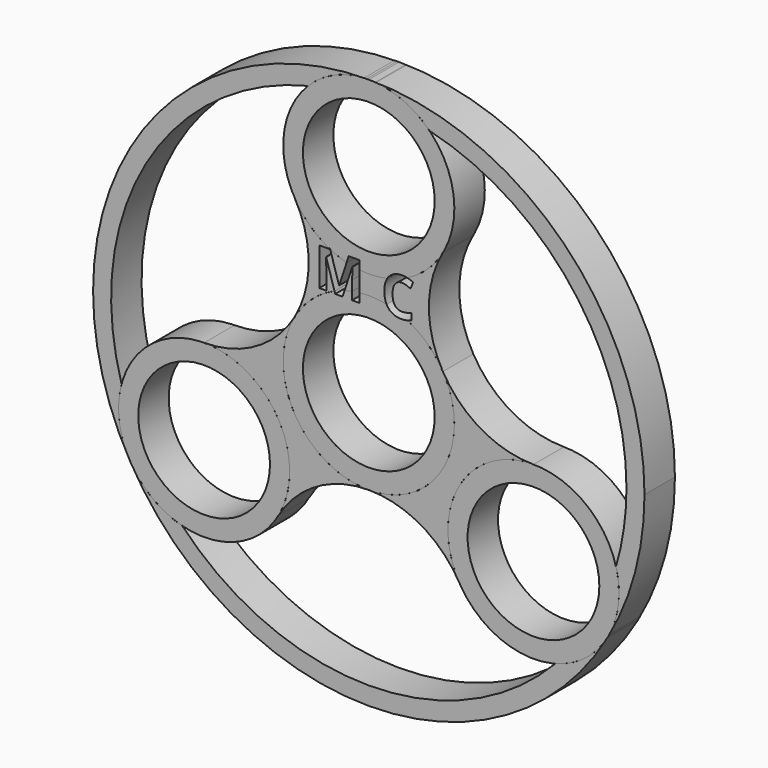
from build123d import *

# Parameters (mm, degrees)
F0_R         = 14.2875
F0_R_2       = 10.9982
F2_DEPTH     = 6.35
F3_TEXT_SIZE = 8.8194444444
F4_DEPTH     = 25.4


# Not quite as in the source:
# - Text() gives the source's letters only with a copy of the font that has no kerning and outlines rounded to 1/6400 em; it was checked with that copy


with BuildPart() as f2:
    # F0 (on Front) → F2 (new body)
    with BuildSketch(Plane.XZ):
        with Locations((0, 31.75)):
            Circle(F0_R)
        with Locations((0, 31.75)):
            Circle(F0_R_2, mode=Mode.SUBTRACT)
    extrude(amount=F2_DEPTH)


with BuildPart() as f2b:
    # F0 (on Front) → F2, piece 2 (new body)
    with BuildSketch(Plane.XZ):
        Circle(F0_R)
        Circle(F0_R_2, mode=Mode.SUBTRACT)
    extrude(amount=F2_DEPTH)


with BuildPart() as f2c:
    # F0 (on Front) → F2, piece 3 (new body)
    with BuildSketch(Plane.XZ):
        with Locations((-27.4963065702, -15.875)):
            Circle(F0_R)
        with Locations((-27.4963065702, -15.875)):
            Circle(F0_R_2, mode=Mode.SUBTRACT)
    extrude(amount=F2_DEPTH)


with BuildPart() as f2d:
    # F0 (on Front) → F2, piece 4 (new body)
    with BuildSketch(Plane.XZ):
        with Locations((27.4963065702, -15.875)):
            Circle(F0_R)
        with Locations((27.4963065702, -15.875)):
            Circle(F0_R_2, mode=Mode.SUBTRACT)
    extrude(amount=F2_DEPTH)


with BuildPart() as f2e:
    # F1 (on Front) → F2, piece 5 (new body)
    with BuildSketch(Plane.XZ):
        with BuildLine():
            ThreePointArc((12.3733379566, 24.60625), (0, 17.4625), (-12.3733379566, 24.60625))
            ThreePointArc((-12.3733379566, 24.60625), (-10.0338065702, 15.8750000272), (-12.3733379294, 7.1437500471))
            ThreePointArc((-12.3733379294, 7.1437500471), (-1.17e-08, 14.2875), (12.3733379177, 7.1437500674))
            ThreePointArc((12.3733379177, 7.1437500674), (10.0338065702, 15.8750000389), (12.3733379566, 24.60625))
        make_face()
    extrude(amount=F2_DEPTH)


with BuildPart() as f2f:
    # F1 (on Front) → F2, piece 6 (new body)
    with BuildSketch(Plane.XZ):
        with BuildLine():
            ThreePointArc((1.61e-08, -14.2875), (-12.3733379662, -7.1437499834), (-12.3733379294, 7.1437500471))
            ThreePointArc((-12.3733379294, 7.1437500471), (-18.7650565466, 0.7520314), (-27.4963065702, -1.5875))
            ThreePointArc((-27.4963065702, -1.5875), (-17.393518434, -5.7722118638), (-13.2088065702, -15.875))
            ThreePointArc((-13.2088065702, -15.875), (-13.6956413271, -19.5728771069), (-15.1229686136, -23.01875))
            ThreePointArc((-15.1229686136, -23.01875), (-8.731249993, -16.6270313824), (1.61e-08, -14.2875))
        make_face()
    extrude(amount=F2_DEPTH)


with BuildPart() as f2g:
    # F1 (on Front) → F2, piece 7 (new body)
    with BuildSketch(Plane.XZ):
        with BuildLine():
            ThreePointArc((27.4963065702, -1.5875), (18.7650565365, 0.7520314059), (12.3733379177, 7.1437500674))
            ThreePointArc((12.3733379177, 7.1437500674), (13.800665233, 3.6978771445), (14.2875, 0))
            ThreePointArc((14.2875, 0), (10.1027881419, -10.1027881305), (1.61e-08, -14.2875))
            ThreePointArc((1.61e-08, -14.2875), (8.731250007, -16.6270313904), (15.1229686136, -23.01875))
            ThreePointArc((15.1229686136, -23.01875), (15.1229686136, -8.73125), (27.4963065702, -1.5875))
        make_face()
    extrude(amount=F2_DEPTH)


with BuildPart() as f2h:
    # F1 (on Front) → F2, piece 8 (new body)
    with BuildSketch(Plane.XZ):
        with BuildLine():
            ThreePointArc((-31.1385341366, -29.6904563661), (-36.1711264704, -27.2275396255), (-39.8696444605, -23.0187501146))
            ThreePointArc((-39.8696444605, -23.0187501146), (0, -46.0375), (39.8696444605, -23.0187501146))
            ThreePointArc((39.8696444605, -23.0187501146), (36.1711264704, -27.2275396255), (31.1385341366, -29.6904563661))
            ThreePointArc((31.1385341366, -29.6904563661), (0, -43.024777831), (-31.1385341366, -29.6904563661))
        make_face()
    extrude(amount=F2_DEPTH)


with BuildPart() as f2i:
    # F1 (on Front) → F2, piece 9 (new body)
    with BuildSketch(Plane.XZ):
        with BuildLine():
            ThreePointArc((-41.2819565313, -12.1215334159), (-37.2605505938, 21.5123889155), (-10.1434223947, 41.811989782))
            ThreePointArc((-10.1434223947, 41.811989782), (-5.4941777093, 44.938884242), (-1.61e-08, 46.0375))
            ThreePointArc((-1.61e-08, 46.0375), (-39.8696445638, 23.0187499357), (-39.8696444605, -23.0187501146))
            ThreePointArc((-39.8696444605, -23.0187501146), (-41.6653042164, -17.7113447254), (-41.2819565313, -12.1215334159))
        make_face()
    extrude(amount=F2_DEPTH)


with BuildPart() as f2j:
    # F1 (on Front) → F2, piece 10 (new body)
    with BuildSketch(Plane.XZ):
        with BuildLine():
            ThreePointArc((46.0375, 0), (32.5534284332, 32.5534284446), (-1.61e-08, 46.0375))
            ThreePointArc((-1.61e-08, 46.0375), (5.4941776945, 44.9388842482), (10.1434223947, 41.811989782))
            ThreePointArc((10.1434223947, 41.811989782), (33.8197427724, 26.5961746538), (43.024777831, 0))
            ThreePointArc((43.024777831, 0), (42.5868437173, -6.1230915075), (41.2819565313, -12.1215334159))
            ThreePointArc((41.2819565313, -12.1215334159), (41.6577883088, -13.9815662898), (41.7838065702, -15.875))
            ThreePointArc((41.7838065702, -15.875), (41.2969717961, -19.5728771708), (39.8696444605, -23.0187501146))
            ThreePointArc((39.8696444605, -23.0187501146), (44.4688102107, -11.9153818528), (46.0375, 0))
        make_face()
    extrude(amount=F2_DEPTH)


with BuildPart() as f4_tool:
    # F3 (on Front) → F4 (new body)
    with BuildSketch(Plane.XZ):
        with Locations((-9.0597963542, 12.7)):
            Text('M', F3_TEXT_SIZE, font='Open Sans', font_style=FontStyle.BOLD, text_align=(TextAlign.LEFT, TextAlign.BOTTOM))
        with Locations((2.0828, 12.7)):
            Text('C', F3_TEXT_SIZE, font='Open Sans', font_style=FontStyle.BOLD, text_align=(TextAlign.LEFT, TextAlign.BOTTOM))
    extrude(amount=F4_DEPTH)


with BuildPart() as f2_1:
    add(f2.part)

    # F4: cut by f4_tool
    add(f4_tool.part, mode=Mode.SUBTRACT)


with BuildPart() as f2b_1:
    add(f2b.part)

    # F4: cut by f4_tool
    add(f4_tool.part, mode=Mode.SUBTRACT)


with BuildPart() as f2e_1:
    add(f2e.part)

    # F4: cut by f4_tool
    add(f4_tool.part, mode=Mode.SUBTRACT)


solid = Compound([f2c.part, f2d.part, f2f.part, f2g.part, f2h.part, f2i.part, f2j.part, f2_1.part, f2b_1.part, f2e_1.part])
